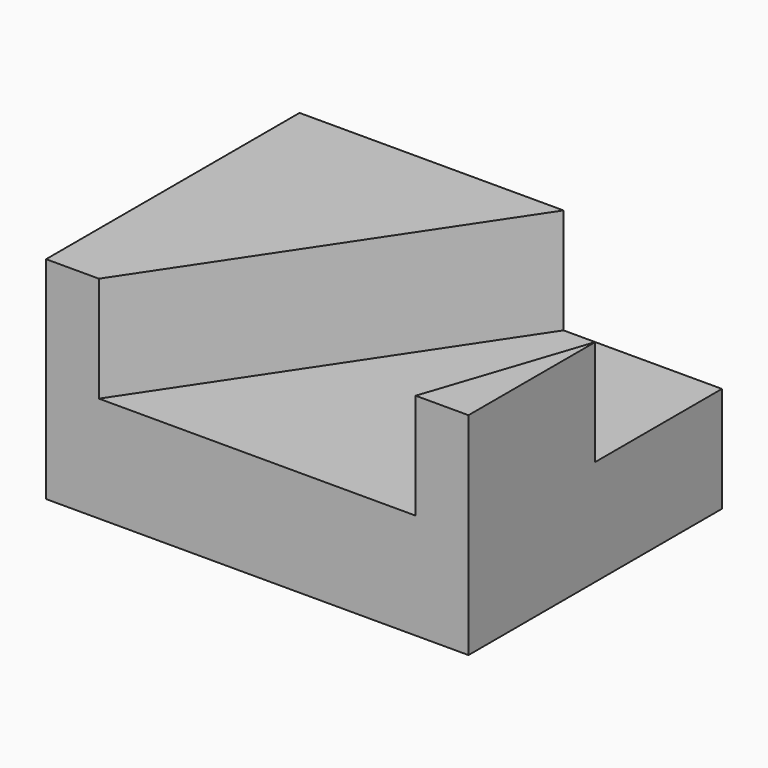
from build123d import *

# Parameters (mm, degrees)
F0_W     = 50.8
F0_H     = 25.4
F1_DEPTH = 38.1
F3_DEPTH = 12.7


# Not quite as in the source:
# - a length typed as a fraction of an inch, garbled in the dataset ("3 / 203.2 mm" for 3/8 in), is restored


with BuildPart() as f1:
    # F0 (on Front) → F1 (new body)
    with BuildSketch(Plane.XZ):
        with Locations((25.4, 12.7)):
            Rectangle(F0_W, F0_H)
    extrude(amount=F1_DEPTH)

    # F2 (on face) → F3 (cut)
    with BuildSketch(Plane.XY.offset(25.4)):
        Polygon((31.75, 0), (6.35, -38.1), (44.45, -38.1), (50.8, -19.05), (50.8, 0), align=None)
    extrude(amount=-F3_DEPTH, mode=Mode.SUBTRACT)


solid = f1.part
